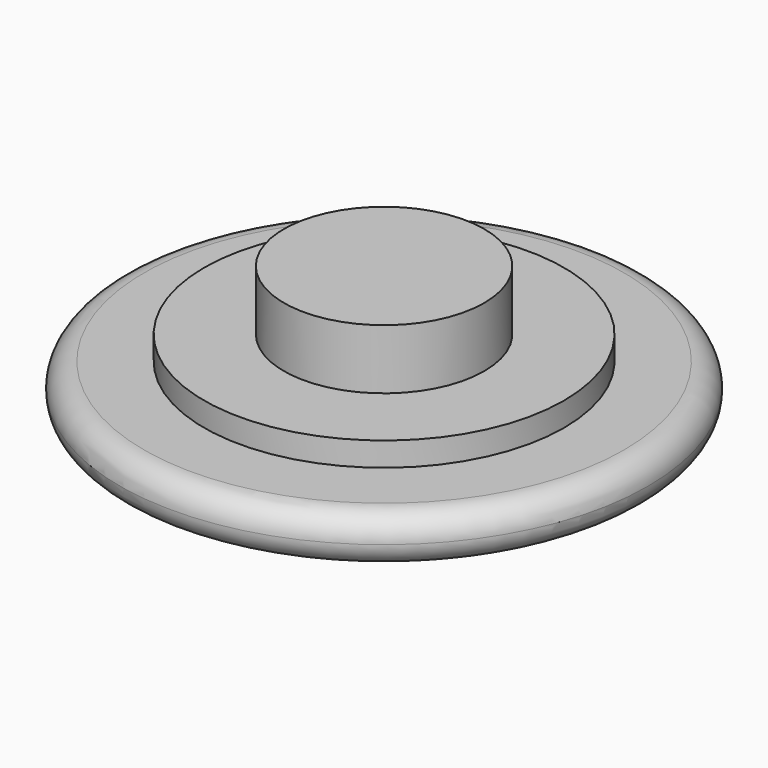
from build123d import *

# Parameters (mm, degrees)
F0_R         = 11
F0_R_2       = 7.5
F1_DEPTH     = 2
F0_R_3       = 4.175
F2_DEPTH     = 3
F3_DEPTH     = 5.5
F4_R         = 0.99999
F5_TEXT_SIZE = 5.529105184
F6_DEPTH     = 1


# Not quite as in the source:
# - a fillet or chamfer is up to 0.001 mm smaller than in the source, because OpenCascade refuses the exact size
# - Text() gives the source's letters only with a copy of the font that has no kerning and outlines rounded to 1/6400 em; it was checked with that copy


with BuildPart() as f1:
    # F0 (on Top) → F1 (new body)
    with BuildSketch(Plane.XY):
        Circle(F0_R)
        Circle(F0_R_2, mode=Mode.SUBTRACT)
    extrude(amount=F1_DEPTH)

    # F0 (on Top) → F2 (join)
    with BuildSketch(Plane.XY):
        Circle(F0_R_2)
        Circle(F0_R_3, mode=Mode.SUBTRACT)
    extrude(amount=F2_DEPTH)

    # F0 (on Top) → F3 (join)
    with BuildSketch(Plane.XY):
        Circle(F0_R_3)
    extrude(amount=F3_DEPTH)

    # F4 (radius 1 in the source; OpenCascade refuses exactly that, so slightly less here)
    f4_edges = [f1.edges().sort_by_distance(p)[0] for p in [
        (-11, 0, 2),
        (-11, 0, 0),
    ]]
    fillet(f4_edges, radius=F4_R)

    # F5 (on face) → F6 (cut)
    with BuildSketch(Plane(origin=(0, 0, 0), x_dir=(1, 0, 0), z_dir=(0, 0, -1))):
        with Locations((-9.892094391, -1.4650831235)):
            Text('Danelle', F5_TEXT_SIZE, font='Open Sans', text_align=(TextAlign.LEFT, TextAlign.BOTTOM))
    extrude(amount=-F6_DEPTH, mode=Mode.SUBTRACT)


solid = f1.part
